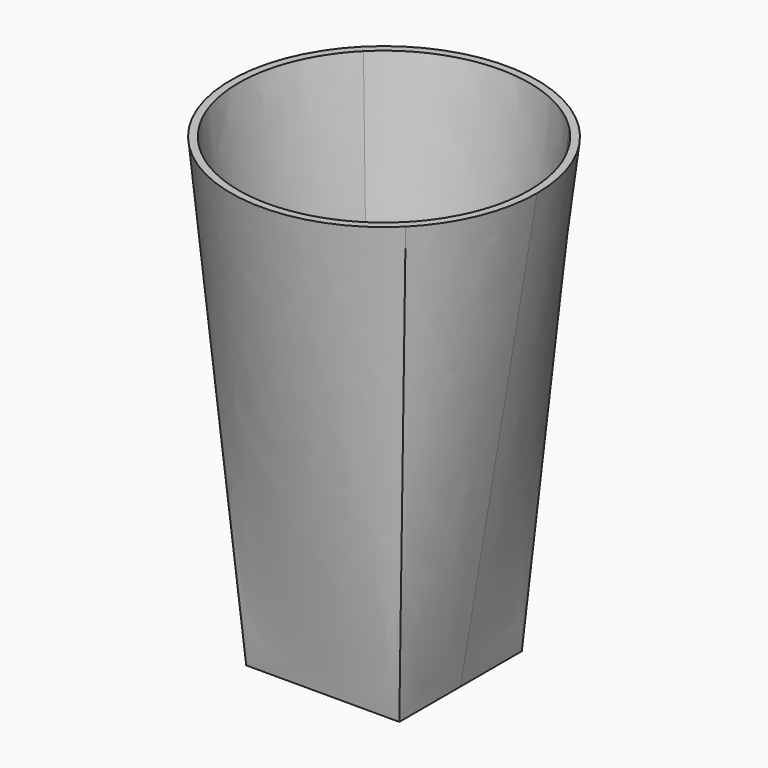
from build123d import *

# Parameters (mm, degrees)
F2_R = 50
F1_W = 50
F1_H = 50
F4_T = 2.5


# Not quite as in the source:
# - a shell that OpenCascade refuses in one call is made with other operations: the cavity is built on its own and cut out


with BuildPart() as f3:
    # F2 (on offset) → F3 section 0
    with BuildSketch(Plane.XY.offset(150)):
        Circle(F2_R)
    # F1 (on Top) → F3 section 1
    with BuildSketch(Plane.XY):
        Rectangle(F1_W, F1_H)
    loft()

    # F4: shell of thickness 2.5, made by hand


with BuildPart() as f4_core1:
    # F4_t2: copy of F3
    add(f3.part)

    # the walls: a layer under each face that stays
    f4_faces = [f4_core1.faces().sort_by_distance(p)[0] for p in [
        (35.5969883078, 15.8170858071, 75),
        (0, 37.4999999981, 75),
        (-37.4999999981, 0, 75),
        (0, -37.4999999981, 75),
        (35.5969883078, -15.8170858071, 75),
        (0, 0, 0),
    ]]
    thicken(f4_faces, amount=-F4_T, mode=Mode.SUBTRACT)


with BuildPart() as f3_1:
    add(f3.part)

    # what is left inside the walls is the cavity
    f4_cavity = [f4_core1.part.solids().sort_by_distance(p)[0] for p in [
        (-39.265085, 0, 100.949484),
    ]]
    add(f4_cavity, mode=Mode.SUBTRACT)


solid = f3_1.part
